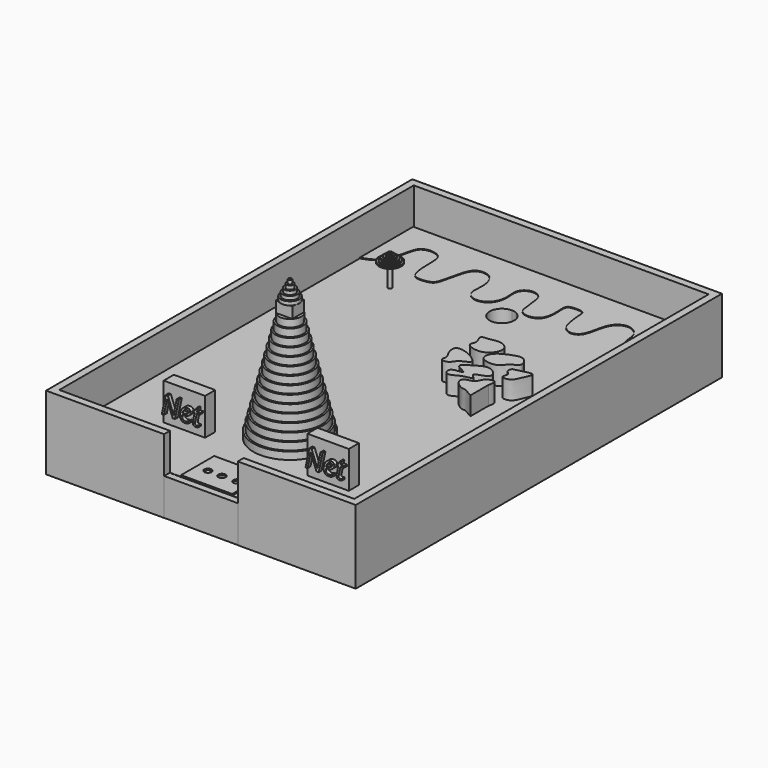
from build123d import *

# Parameters (mm, degrees)
F0_W          = 50.8
F0_H          = 76.2
F1_DEPTH      = 12.7
F2_R          = 12.7
F3_DEPTH      = 2.54
F4_R          = 12.065
F5_DEPTH      = 2.54
F6_R          = 11.43
F7_DEPTH      = 2.54
F8_R          = 10.795
F9_DEPTH      = 2.54
F10_R         = 10.16
F11_DEPTH     = 2.54
F12_R         = 9.525
F13_DEPTH     = 2.54
F14_R         = 8.89
F15_DEPTH     = 2.54
F16_R         = 8.255
F17_DEPTH     = 2.54
F18_R         = 7.62
F19_DEPTH     = 2.54
F20_R         = 6.985
F21_DEPTH     = 2.54
F22_R         = 6.35
F23_DEPTH     = 2.54
F24_R         = 5.715
F25_DEPTH     = 2.54
F26_R         = 5.08
F27_DEPTH     = 2.54
F28_R         = 4.445
F29_DEPTH     = 2.54
F30_R         = 3.81
F31_DEPTH     = 2.54
F33_W         = 5.6803734042
F33_H         = 5.0760805607
F34_DEPTH     = 3.81
F35_R         = 3.175
F36_DEPTH     = 1.27
F37_R         = 2.54
F38_DEPTH     = 1.27
F39_R         = 1.905
F40_DEPTH     = 1.27
F41_R         = 1.27
F42_DEPTH     = 1.27
F43_R         = 0.635
F44_DEPTH     = 1.27
F46_DEPTH     = 0.254
F47_DEPTH     = 6.35
F48_W         = 14.2592061311
F48_H         = 4.3719261885
F49_DEPTH     = 12.7
F50_TEXT_SIZE = 8.8181388771
F51_DEPTH     = 1.27
F52_W         = 14.2592044
F52_H         = 4.3719261885
F53_DEPTH     = 12.7
F54_TEXT_SIZE = 8.8181378066
F55_DEPTH     = 1.27
F57_DEPTH     = 6.35
F59_DEPTH     = 6.35
F60_W         = 101.6
F60_H         = 2.54
F60_W_2       = 38.1
F61_DEPTH     = 25.4
F62_W         = 17.5981968641
F62_H         = 14.2608052015
F62_R         = 1.27
F63_DEPTH     = 0.508
F64_R         = 0.635
F65_DEPTH     = 7.62
F66_R         = 3.81
F67_DEPTH     = 0.508
F68_R         = 3.175
F69_DEPTH     = 0.508
F70_R         = 2.54
F71_DEPTH     = 0.508
F72_R         = 1.905
F73_DEPTH     = 0.508
F74_R         = 1.27
F75_DEPTH     = 0.508
F76_R         = 0.635
F77_DEPTH     = 0.508
F78_W         = 25.4
F78_H         = 2.3591564351
F79_DEPTH     = 12.7


# Not quite as in the source:
# - a feature names something its author has since deleted; it is built from what else it names
# - Text() gives the source's letters only with a copy of the font that has no kerning and outlines rounded to 1/6400 em; it was checked with that copy


with BuildPart() as f1:
    # F0 (on Top) → F1 (new body)
    with BuildSketch(Plane.XY):
        with Locations((-25.4, -38.1)):
            Rectangle(F0_W, F0_H)
        with Locations((25.4, -38.1)):
            Rectangle(F0_W, F0_H)
        with BuildLine():
            Line((-50.8, 0), (0, 0))
            Line((0, 0), (0, 46.6641196469))
            ThreePointArc((0, 46.6641196469), (-4.2333333333, 50.8974529803), (0, 55.1307863136))
            Line((0, 55.1307863136), (0, 76.2))
            Line((0, 76.2), (-50.8, 76.2))
            Line((-50.8, 76.2), (-50.8, 0))
        make_face()
        with BuildLine():
            Line((0, 46.6641196469), (0, 0))
            Line((0, 0), (50.8, 0))
            Line((50.8, 0), (50.8, 76.2))
            Line((50.8, 76.2), (0, 76.2))
            Line((0, 76.2), (0, 55.1307863136))
            ThreePointArc((0, 55.1307863136), (2.993418707, 53.8908716873), (4.2333333333, 50.8974529803))
            ThreePointArc((4.2333333333, 50.8974529803), (2.993418707, 47.9040342733), (0, 46.6641196469))
        make_face()
    extrude(amount=F1_DEPTH)

    # F2 (on face) → F3 (join)
    with BuildSketch(Plane.XY.offset(12.7)):
        with Locations((0, -40.3213936513)):
            Circle(F2_R)
    extrude(amount=F3_DEPTH)

    # F4 (on face) → F5 (join)
    with BuildSketch(Plane.XY.offset(15.24)):
        with Locations((0, -40.3213936513)):
            Circle(F4_R)
    extrude(amount=F5_DEPTH)

    # F6 (on face) → F7 (join)
    with BuildSketch(Plane.XY.offset(17.78)):
        with Locations((0, -40.3213936513)):
            Circle(F6_R)
    extrude(amount=F7_DEPTH)

    # F8 (on face) → F9 (join)
    with BuildSketch(Plane.XY.offset(20.32)):
        with Locations((0, -40.3213936513)):
            Circle(F8_R)
    extrude(amount=F9_DEPTH)

    # F10 (on face) → F11 (join)
    with BuildSketch(Plane.XY.offset(22.86)):
        with Locations((0, -40.3213936513)):
            Circle(F10_R)
    extrude(amount=F11_DEPTH)

    # F12 (on face) → F13 (join)
    with BuildSketch(Plane.XY.offset(25.4)):
        with Locations((0, -40.3213936513)):
            Circle(F12_R)
    extrude(amount=F13_DEPTH)

    # F14 (on face) → F15 (join)
    with BuildSketch(Plane.XY.offset(27.94)):
        with Locations((0, -40.3213936513)):
            Circle(F14_R)
    extrude(amount=F15_DEPTH)

    # F16 (on face) → F17 (join)
    with BuildSketch(Plane.XY.offset(30.48)):
        with Locations((0, -40.3213936513)):
            Circle(F16_R)
    extrude(amount=F17_DEPTH)

    # F18 (on face) → F19 (join)
    with BuildSketch(Plane.XY.offset(33.02)):
        with Locations((0, -40.3213936513)):
            Circle(F18_R)
    extrude(amount=F19_DEPTH)

    # F20 (on face) → F21 (join)
    with BuildSketch(Plane.XY.offset(35.56)):
        with Locations((0, -40.3213936513)):
            Circle(F20_R)
    extrude(amount=F21_DEPTH)

    # F22 (on face) → F23 (join)
    with BuildSketch(Plane.XY.offset(38.1)):
        with Locations((0, -40.3213936513)):
            Circle(F22_R)
    extrude(amount=F23_DEPTH)

    # F24 (on face) → F25 (join)
    with BuildSketch(Plane.XY.offset(40.64)):
        with Locations((0, -40.3213936513)):
            Circle(F24_R)
    extrude(amount=F25_DEPTH)

    # F26 (on face) → F27 (join)
    with BuildSketch(Plane.XY.offset(43.18)):
        with Locations((0, -40.3213936513)):
            Circle(F26_R)
    extrude(amount=F27_DEPTH)

    # F28 (on face) → F29 (join)
    with BuildSketch(Plane.XY.offset(45.72)):
        with Locations((0, -40.3213936513)):
            Circle(F28_R)
    extrude(amount=F29_DEPTH)

    # F30 (on face) → F31 (join)
    with BuildSketch(Plane.XY.offset(48.26)):
        with Locations((0, -40.3213936513)):
            Circle(F30_R)
    extrude(amount=F31_DEPTH)

    # F33 (on face) → F34 (join)
    with BuildSketch(Plane.XY.offset(50.8)):
        with Locations((-0.0593231525, -40.3204448521)):
            Rectangle(F33_W, F33_H)
    extrude(amount=F34_DEPTH)

    # F35 (on face) → F36 (join)
    with BuildSketch(Plane.XY.offset(54.61)):
        with Locations((0, -40.3632596135)):
            Circle(F35_R)
    extrude(amount=F36_DEPTH)

    # F37 (on face) → F38 (join)
    with BuildSketch(Plane.XY.offset(55.88)):
        with Locations((0, -40.3632596135)):
            Circle(F37_R)
    extrude(amount=F38_DEPTH)

    # F39 (on face) → F40 (join)
    with BuildSketch(Plane.XY.offset(57.15)):
        with Locations((0, -40.3632596135)):
            Circle(F39_R)
    extrude(amount=F40_DEPTH)

    # F41 (on face) → F42 (join)
    with BuildSketch(Plane.XY.offset(58.42)):
        with Locations((0, -40.3632596135)):
            Circle(F41_R)
    extrude(amount=F42_DEPTH)

    # F43 (on face) → F44 (join)
    with BuildSketch(Plane.XY.offset(59.69)):
        with Locations((0, -40.3632596135)):
            Circle(F43_R)
    extrude(amount=F44_DEPTH)

    # F45 (on face) → F46 (join)
    with BuildSketch(Plane.XY.offset(12.7)):
        with BuildLine():
            Line((-50.8, 76.2), (-50.8, 53.1264543533))
            add(Edge.make_bspline(
                [(-50.8, 53.1264543533), (-49.1404273386, 53.7261613802), (-45.8765340753, 54.9056094214), (-43.7674298873, 59.4610029171), (-42.6251788822, 63.8987785589), (-41.820770591, 67.8088848575), (-37.8239583442, 68.511250669), (-35.3904996184, 67.5426139949), (-33.8735159329, 65.9655808334), (-34.0676818764, 60.7001757557), (-33.8447902415, 58.2824455432), (-33.1966856986, 53.3818261331), (-28.9161354004, 53.5017081487), (-25.7660173763, 54.2362699759), (-25.0317137871, 58.0701666465), (-24.3193942393, 60.8986992391), (-23.6022658779, 64.210216286), (-21.919734242, 67.3897768805), (-18.2590473813, 67.4581168835), (-16.1041663507, 66.0393218919), (-14.7639546298, 63.2991814448), (-14.5533272132, 59.6545249884), (-15.1920008355, 55.9423270865), (-12.3519748454, 53.2501404133), (-8.5124699015, 53.7080955929), (-5.8482457883, 56.5216565258), (-5.346446833, 60.7997074287), (-6.1305777909, 64.8946330577), (-2.4830735424, 67.4808526668), (1.2476934043, 65.8798746993), (1.6846090391, 62.9708552919), (2.2402475012, 59.3026013165), (2.3369741552, 56.159072675), (5.0135377235, 54.5433778217), (8.9162573988, 55.358853461), (10.4003242923, 58.5507534179), (10.3904989905, 62.5409573397), (10.0205470635, 66.0476543095), (13.0899796438, 66.367844594), (16.4674346472, 66.2116127845), (16.2449679372, 62.8268710613), (16.8250368654, 59.2790773901), (17.5984687287, 55.7363250052), (20.8192249532, 53.9541591142), (23.8006814067, 55.3874777639), (24.7722862833, 58.8166719493), (25.2520174936, 61.4036865011), (26.3919972503, 65.5828233368), (30.7977355767, 67.901632876), (35.4694475107, 64.6923747516), (35.1426484522, 59.8298776894), (37.0071216479, 55.9985398293), (40.1368596239, 52.8215190771), (43.8780425684, 56.775004683), (45.0702500011, 60.7924588874), (45.1702474732, 63.0124679443), (46.5212655601, 66.2951052792), (49.2077608966, 66.1112705809), (50.7120991999, 63.5231725093), (50.8, 63.2106214762)],
                knots=[0, 0, 0, 0, 0.0212502508, 0.0417930183, 0.0623992021, 0.08024358, 0.0979189514, 0.112918674, 0.1262272693, 0.1472448811, 0.1632560223, 0.18229659, 0.2002370675, 0.2165251655, 0.2341452845, 0.2506563636, 0.2680872708, 0.2852123589, 0.3021090267, 0.3169208542, 0.3329899062, 0.3511487514, 0.3690346577, 0.3862183497, 0.4038829865, 0.4217826714, 0.4412306939, 0.4598555674, 0.4778912741, 0.4953148199, 0.510948098, 0.5293995923, 0.5456186598, 0.5610840346, 0.5789422985, 0.5958675172, 0.6151937209, 0.631286497, 0.6464724026, 0.6624212536, 0.6780390081, 0.6964905022, 0.7141515669, 0.730949226, 0.7468980734, 0.7641781461, 0.7798525608, 0.7989901943, 0.8185234598, 0.8389283151, 0.8591185028, 0.8788576024, 0.8963405132, 0.9162642368, 0.9357443621, 0.9501447763, 0.966708704, 0.9807168691, 0.9970195422, 0.9970195422, 0.9970195422, 0.9970195422], degree=3))
            Line((50.8, 63.2106214762), (50.8, 76.2))
            Line((50.8, 76.2), (-50.8, 76.2))
        make_face()
    extrude(amount=F46_DEPTH)

    # F0 (on Top) → F47 (join)
    with BuildSketch(Plane.XY):
        with BuildLine():
            ThreePointArc((0, 55.1307863136), (-4.2333333333, 50.8974529803), (0, 46.6641196469))
            Line((0, 46.6641196469), (0, 55.1307863136))
        make_face()
        with BuildLine():
            Line((0, 55.1307863136), (0, 46.6641196469))
            ThreePointArc((0, 46.6641196469), (2.993418707, 47.9040342733), (4.2333333333, 50.8974529803))
            ThreePointArc((4.2333333333, 50.8974529803), (2.993418707, 53.8908716873), (0, 55.1307863136))
        make_face()
    extrude(amount=F47_DEPTH)

    # F48 (on face) → F49 (join)
    with BuildSketch(Plane.XY.offset(12.7)):
        with Locations((-25.1516578719, -52.2259883583)):
            Rectangle(F48_W, F48_H)
    extrude(amount=F49_DEPTH)

    # F50 (on face) → F51 (join)
    with BuildSketch(Plane.XZ.offset(54.4119514525)):
        with Locations((-32.2812609375, 15.8318612551)):
            Text('Net', F50_TEXT_SIZE, font='Open Sans', font_style=FontStyle.ITALIC, text_align=(TextAlign.LEFT, TextAlign.BOTTOM))
    extrude(amount=F51_DEPTH)

    # F52 (on face) → F53 (join)
    with BuildSketch(Plane.XY.offset(12.7)):
        with Locations((24.3594777497, -52.2259883583)):
            Rectangle(F52_W, F52_H)
    extrude(amount=F53_DEPTH)

    # F54 (on face) → F55 (join)
    with BuildSketch(Plane.XZ.offset(54.4119514525)):
        with Locations((17.2298755497, 15.7736718567)):
            Text('Net', F54_TEXT_SIZE, font='Open Sans', font_style=FontStyle.ITALIC, text_align=(TextAlign.LEFT, TextAlign.BOTTOM))
    extrude(amount=F55_DEPTH)

    # F56 (on face) → F57 (join)
    with BuildSketch(Plane.XY.offset(12.7)):
        with BuildLine():
            Line((29.9047287554, 0), (29.9047287554, 7.7237379737))
            add(Edge.make_bspline(
                [(29.9047287554, 0), (28.4243061964, 0.846996038), (26.3722954666, 2.0210155419), (25.7528726234, 1.5440521884), (22.3129411796, 3.4139806169), (21.9359434701, 6.5389103006), (26.2218293607, 6.5065948247), (26.6522833606, 10.0657353607), (30.6770673499, 11.002400815), (30.1610594214, 8.8118900298), (29.9047287554, 7.7237379737)],
                knots=[0, 0, 0, 0, 0.1544707926, 0.2141116548, 0.3603137356, 0.4747523513, 0.6131544753, 0.7500747384, 0.8758478209, 1, 1, 1, 1], degree=3))
        make_face()
    extrude(amount=F57_DEPTH)

    # F58 (on face) → F59 (join)
    with BuildSketch(Plane.XY.offset(12.7)):
        with BuildLine():
            add(Edge.make_bspline(
                [(21.1907681078, 7.327648811), (19.4816179622, 6.7387774734), (16.9745449473, 4.5024432322), (15.1040723558, 9.299994493), (22.6963371152, 8.7512977325), (14.8042168908, 11.4954507355), (19.6731404612, 14.0072018295), (24.0481845418, 16.9912437944), (29.2988191549, 11.2842804114), (21.055184284, 10.4499669902), (25.5805315689, 7.8329219226), (22.6352632711, 7.8253358055), (21.1907681078, 7.327648811)],
                knots=[0, 0, 0, 0, 0.1098552575, 0.1919744414, 0.2928946392, 0.3957808427, 0.4919686298, 0.6137496957, 0.7217657224, 0.8333187482, 0.9071553845, 1, 1, 1, 1], degree=3))
        make_face()
        with BuildLine():
            add(Edge.make_bspline(
                [(29.9047287554, 13.8631183654), (30.2013986606, 13.3298866541), (33.2785066816, 13.4335557698), (34.1478939356, 16.7815740252), (36.7526226309, 21.2958727288), (30.4022649705, 18.9368113574), (29.0001062871, 19.1962326304), (28.4618680241, 16.940195425), (30.7965700149, 16.1280713189), (29.6438839674, 14.3319583462), (29.9047287554, 13.8631183654)],
                knots=[0, 0, 0, 0, 0.1262178262, 0.2782765704, 0.4162048521, 0.5888798728, 0.6833331872, 0.7827311863, 0.8890239235, 1, 1, 1, 1], degree=3))
        make_face()
        with BuildLine():
            add(Edge.make_bspline(
                [(24.3594814092, 18.2201005518), (25.5673387802, 18.7388613758), (26.5067397879, 20.9213988724), (29.5521223834, 21.6050772546), (29.3891323235, 24.1532461924), (27.1659954716, 26.2572545542), (24.290308705, 25.3733225648), (20.4411063508, 23.86651669), (18.4988402734, 21.3713244317), (18.7673034994, 18.1356523073), (22.9185212883, 17.6012247826), (24.3594814092, 18.2201005518)],
                knots=[0, 0, 0, 0, 0.1188151489, 0.2208146205, 0.3101422085, 0.4137531204, 0.5199821536, 0.6495034979, 0.7589070135, 0.8582548773, 1, 1, 1, 1], degree=3))
        make_face()
        with BuildLine():
            add(Edge.make_bspline(
                [(13.4670296684, 18.814234063), (15.5945116725, 17.9994807373), (19.8609655596, 15.1489063172), (14.4176375206, 14.0655634853), (13.6755782317, 11.0927011225), (10.2117953168, 11.0370923734), (11.3110982623, 13.5209383561), (9.7134526639, 15.2109528066), (8.5737507848, 19.7382661179), (11.6626166643, 19.5052629381), (13.4670296684, 18.814234063)],
                knots=[0, 0, 0, 0, 0.1668080505, 0.2958681724, 0.4178429798, 0.5227654545, 0.61767137, 0.7276378588, 0.8585226033, 1, 1, 1, 1], degree=3))
        make_face()
        with BuildLine():
            add(Edge.make_bspline(
                [(11.2885385752, 22.9731686413), (11.7368120378, 21.968507128), (17.6286597506, 20.1636515153), (21.5342775366, 26.8405942307), (16.7095594392, 29.7723345998), (13.8382433701, 28.4844399554), (9.7275994012, 28.7680695089), (12.5179884188, 25.0567590992), (11.0084359837, 23.6009289638), (11.2885385752, 22.9731686413)],
                knots=[0, 0, 0, 0, 0.1763982627, 0.353438365, 0.5031095232, 0.6394917207, 0.7598970915, 0.8897779712, 1, 1, 1, 1], degree=3))
        make_face()
    extrude(amount=F59_DEPTH)

    # F60 (on Top) → F61 (join)
    with BuildSketch(Plane.XY):
        with Locations((0, 77.6955449176)):
            Rectangle(F60_W, F60_H)
        Polygon((-50.8, -76.2), (-50.8, 76.4255449176), (-50.8, 78.9655449176), (-53.34, 78.9655449176), (-53.34, -78.74), (-50.8, -78.74), align=None)
        Polygon((50.8, 76.4255449176), (50.8, -76.2), (50.8, -78.74), (53.34, -78.74), (53.34, 78.9655449176), (50.8, 78.9655449176), align=None)
        with Locations((-31.75, -77.47)):
            Rectangle(F60_W_2, F60_H)
        with Locations((31.75, -77.47)):
            Rectangle(F60_W_2, F60_H)
    extrude(amount=F61_DEPTH)

    # F62 (on face) → F63 (join)
    with BuildSketch(Plane.XY.offset(12.7)):
        with Locations((-0.06688945, -69.0695973992)):
            Rectangle(F62_W, F62_H)
        with Locations((-4.8164324835, -69.6759074926)):
            Circle(F62_R, mode=Mode.SUBTRACT)
        with Locations((0, -69.6759074926)):
            Circle(F62_R, mode=Mode.SUBTRACT)
        with Locations((5.1648365334, -69.6759074926)):
            Circle(F62_R, mode=Mode.SUBTRACT)
    extrude(amount=F63_DEPTH)

    # F64 (on face) → F65 (join)
    with BuildSketch(Plane.XY.offset(12.7)):
        with Locations((-33.814959228, 44.994443655)):
            Circle(F64_R)
    extrude(amount=F65_DEPTH)

    # F66 (on face) → F67 (join)
    with BuildSketch(Plane.XY.offset(20.32)):
        with Locations((-33.814959228, 44.994443655)):
            Circle(F66_R)
    extrude(amount=F67_DEPTH)

    # F68 (on face) → F69 (join)
    with BuildSketch(Plane.XY.offset(20.828)):
        with Locations((-33.814959228, 44.994443655)):
            Circle(F68_R)
    extrude(amount=F69_DEPTH)

    # F70 (on face) → F71 (join)
    with BuildSketch(Plane.XY.offset(21.336)):
        with Locations((-33.814959228, 44.994443655)):
            Circle(F70_R)
    extrude(amount=F71_DEPTH)

    # F72 (on face) → F73 (join)
    with BuildSketch(Plane.XY.offset(21.844)):
        with Locations((-33.814959228, 44.994443655)):
            Circle(F72_R)
    extrude(amount=F73_DEPTH)

    # F74 (on face) → F75 (join)
    with BuildSketch(Plane.XY.offset(22.352)):
        with Locations((-33.814959228, 44.994443655)):
            Circle(F74_R)
    extrude(amount=F75_DEPTH)

    # F76 (on face) → F77 (join)
    with BuildSketch(Plane.XY.offset(22.86)):
        with Locations((-33.814959228, 44.994443655)):
            Circle(F76_R)
    extrude(amount=F77_DEPTH)

    # F78 (on Top) → F79 (join)
    with BuildSketch(Plane.XY):
        with Locations((-0.0214525498, -77.5076858699)):
            Rectangle(F78_W, F78_H)
    extrude(amount=F79_DEPTH)


solid = f1.part
